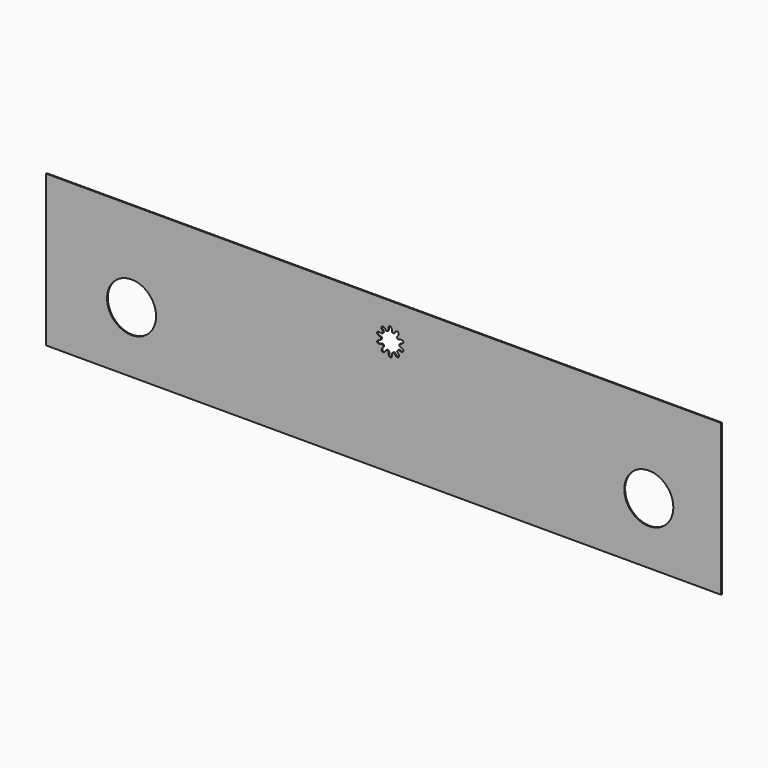
from build123d import *

# Parameters (mm, degrees)
F0_W     = 89.1250632703
F0_H     = 19.9663289823
F0_R     = 3.235221554
F1_DEPTH = 0.127


# Not quite as in the source:
# - ends of sketch curves that miss each other by under 0.0002 mm in the source are joined


with BuildPart() as f1:
    # F0 (on Front) → F1 (new body)
    with BuildSketch(Plane.XZ):
        with Locations((-0.8681025356, -5.2086075302)):
            Rectangle(F0_W, F0_H)
        with Locations((-34.1453179717, -7.0894937962)):
            Circle(F0_R, mode=Mode.SUBTRACT)
        with Locations((34.1453179717, -7.0894937962)):
            Circle(F0_R, mode=Mode.SUBTRACT)
        with BuildLine():
            Line((0.638931, 1.307427), (0.642386, 1.31177))
            Line((0.642386, 1.31177), (0.645946, 1.316251))
            Line((0.645946, 1.316251), (0.649602, 1.320915))
            Line((0.649602, 1.320915), (0.653347, 1.325811))
            Line((0.653347, 1.325811), (0.657176, 1.330987))
            Line((0.657176, 1.330987), (0.66108, 1.336491))
            Line((0.66108, 1.336491), (0.665063, 1.34235))
            Line((0.665063, 1.34235), (0.66917, 1.34852))
            Line((0.66917, 1.34852), (0.673459, 1.354933))
            Line((0.673459, 1.354933), (0.677985, 1.361525))
            Line((0.677985, 1.361525), (0.682804, 1.368231))
            Line((0.682804, 1.368231), (0.687974, 1.374984))
            Line((0.687974, 1.374984), (0.693549, 1.38172))
            Line((0.693549, 1.38172), (0.699587, 1.388373))
            Line((0.699587, 1.388373), (0.706145, 1.394901))
            Line((0.706145, 1.394901), (0.713282, 1.401347))
            Line((0.713282, 1.401347), (0.721059, 1.407781))
            Line((0.721059, 1.407781), (0.729537, 1.41427))
            Line((0.729537, 1.41427), (0.738776, 1.420881))
            Line((0.738776, 1.420881), (0.748838, 1.427684))
            Line((0.748838, 1.427684), (0.759782, 1.434744))
            Line((0.759782, 1.434744), (0.771669, 1.44213))
            Line((0.771669, 1.44213), (0.784656, 1.449932))
            Line((0.784656, 1.449932), (0.799284, 1.458325))
            Line((0.799284, 1.458325), (0.816191, 1.467508))
            Line((0.816191, 1.467508), (0.836013, 1.477679))
            Line((0.836013, 1.477679), (0.859387, 1.489035))
            Line((0.859387, 1.489035), (0.886951, 1.501775))
            Line((0.886951, 1.501775), (0.919341, 1.516097))
            Line((0.919341, 1.516097), (0.949649, 1.528989))
            ThreePointArc((0.949649, 1.528989), (1.0419801318, 1.4676230494), (1.1303581966, 1.4006892437))
            Line((1.1303581966, 1.4006892437), (1.128181, 1.367826))
            Line((1.128181, 1.367826), (1.12534, 1.332524))
            Line((1.12534, 1.332524), (1.122401, 1.302301))
            Line((1.122401, 1.302301), (1.119386, 1.27649))
            Line((1.119386, 1.27649), (1.11632, 1.254423))
            Line((1.11632, 1.254423), (1.113225, 1.235434))
            Line((1.113225, 1.235434), (1.110125, 1.218856))
            Line((1.110125, 1.218856), (1.107041, 1.204023))
            Line((1.107041, 1.204023), (1.103988, 1.190365))
            Line((1.103988, 1.190365), (1.100931, 1.177705))
            Line((1.100931, 1.177705), (1.097827, 1.165964))
            Line((1.097827, 1.165964), (1.094631, 1.155061))
            Line((1.094631, 1.155061), (1.091301, 1.144918))
            Line((1.091301, 1.144918), (1.087791, 1.135454))
            Line((1.087791, 1.135454), (1.084058, 1.126591))
            Line((1.084058, 1.126591), (1.080058, 1.118248))
            Line((1.080058, 1.118248), (1.075768, 1.110353))
            Line((1.075768, 1.110353), (1.071247, 1.102868))
            Line((1.071247, 1.102868), (1.066576, 1.095761))
            Line((1.066576, 1.095761), (1.061834, 1.089))
            Line((1.061834, 1.089), (1.057103, 1.082554))
            Line((1.057103, 1.082554), (1.052463, 1.07639))
            Line((1.052463, 1.07639), (1.047993, 1.070478))
            Line((1.047993, 1.070478), (1.043774, 1.064786))
            Line((1.043774, 1.064786), (1.039866, 1.059286))
            Line((1.039866, 1.059286), (1.036242, 1.053965))
            Line((1.036242, 1.053965), (1.032854, 1.048814))
            Line((1.032854, 1.048814), (1.029656, 1.043825))
            Line((1.029656, 1.043825), (1.0266, 1.038987))
            Line((1.0266, 1.038987), (1.023639, 1.034293))
            Line((1.023639, 1.034293), (1.020725, 1.029733))
            Line((1.020725, 1.029733), (1.017811, 1.025298))
            Line((1.017811, 1.025298), (1.014863, 1.020986))
            Line((1.014863, 1.020986), (1.011898, 1.016826))
            Line((1.011898, 1.016826), (1.008947, 1.012851))
            Line((1.008947, 1.012851), (1.00604, 1.009097))
            Line((1.00604, 1.009097), (1.003207, 1.005598))
            Line((1.003207, 1.005598), (1.00048, 1.00239))
            Line((1.00048, 1.00239), (0.997889, 0.999506))
            Line((0.997889, 0.999506), (0.995464, 0.996983))
            Line((0.995464, 0.996983), (0.918412, 0.888456))
            ThreePointArc((0.918412, 0.888456), (0.900022697, 0.8267789399), (0.9230261025, 0.7666700851))
            ThreePointArc((0.9230261025, 0.7666700851), (0.9629750976, 0.7158484276), (1.0001292142, 0.662949142))
            ThreePointArc((1.0001292142, 0.662949142), (1.0510595113, 0.6236013113), (1.115418799, 0.6234375965))
            Line((1.115418799, 0.6234375965), (1.241546, 0.665948))
            Line((1.241546, 0.665948), (1.244661, 0.667543))
            Line((1.244661, 0.667543), (1.248169, 0.669193))
            Line((1.248169, 0.669193), (1.252027, 0.67088))
            Line((1.252027, 0.67088), (1.256194, 0.672584))
            Line((1.256194, 0.672584), (1.260626, 0.674286))
            Line((1.260626, 0.674286), (1.265283, 0.675967))
            Line((1.265283, 0.675967), (1.270122, 0.677607))
            Line((1.270122, 0.677607), (1.2751, 0.679188))
            Line((1.2751, 0.679188), (1.280186, 0.6807))
            Line((1.280186, 0.6807), (1.285393, 0.682176))
            Line((1.285393, 0.682176), (1.290741, 0.683659))
            Line((1.290741, 0.683659), (1.296254, 0.685192))
            Line((1.296254, 0.685192), (1.301953, 0.686816))
            Line((1.301953, 0.686816), (1.307862, 0.688576))
            Line((1.307862, 0.688576), (1.314001, 0.690513))
            Line((1.314001, 0.690513), (1.320394, 0.692671))
            Line((1.320394, 0.692671), (1.327061, 0.69507))
            Line((1.327061, 0.69507), (1.33401, 0.697647))
            Line((1.33401, 0.697647), (1.341249, 0.700315))
            Line((1.341249, 0.700315), (1.348786, 0.702987))
            Line((1.348786, 0.702987), (1.356626, 0.70558))
            Line((1.356626, 0.70558), (1.364778, 0.708005))
            Line((1.364778, 0.708005), (1.373248, 0.710177))
            Line((1.373248, 0.710177), (1.382044, 0.71201))
            Line((1.382044, 0.71201), (1.391186, 0.713437))
            Line((1.391186, 0.713437), (1.400749, 0.714457))
            Line((1.400749, 0.714457), (1.410822, 0.715091))
            Line((1.410822, 0.715091), (1.421495, 0.715357))
            Line((1.421495, 0.715357), (1.432856, 0.715275))
            Line((1.432856, 0.715275), (1.444994, 0.714864))
            Line((1.444994, 0.714864), (1.457998, 0.714144))
            Line((1.457998, 0.714144), (1.471956, 0.713132))
            Line((1.471956, 0.713132), (1.487049, 0.71181))
            Line((1.487049, 0.71181), (1.503817, 0.710002))
            Line((1.503817, 0.710002), (1.522892, 0.707494))
            Line((1.522892, 0.707494), (1.544906, 0.704071))
            Line((1.544906, 0.704071), (1.570492, 0.69952))
            Line((1.570492, 0.69952), (1.60028, 0.693625))
            Line((1.60028, 0.693625), (1.634903, 0.686173))
            Line((1.634903, 0.686173), (1.666999, 0.678788))
            ThreePointArc((1.666999, 0.678788), (1.7056267642, 0.5748715955), (1.7377833197, 0.4687740862))
            Line((1.7377833197, 0.4687740862), (1.716705, 0.443466))
            Line((1.716705, 0.443466), (1.693657, 0.416577))
            Line((1.693657, 0.416577), (1.673515, 0.393853))
            Line((1.673515, 0.393853), (1.655905, 0.374743))
            Line((1.655905, 0.374743), (1.640453, 0.358693))
            Line((1.640453, 0.358693), (1.626788, 0.34515))
            Line((1.626788, 0.34515), (1.614536, 0.33356))
            Line((1.614536, 0.33356), (1.603322, 0.323372))
            Line((1.603322, 0.323372), (1.592824, 0.314118))
            Line((1.592824, 0.314118), (1.58291, 0.305672))
            Line((1.58291, 0.305672), (1.573497, 0.297998))
            Line((1.573497, 0.297998), (1.564503, 0.291056))
            Line((1.564503, 0.291056), (1.555847, 0.284807))
            Line((1.555847, 0.284807), (1.547445, 0.279214))
            Line((1.547445, 0.279214), (1.539215, 0.274237))
            Line((1.539215, 0.274237), (1.531075, 0.269839))
            Line((1.531075, 0.269839), (1.522964, 0.265974))
            Line((1.522964, 0.265974), (1.514907, 0.262576))
            Line((1.514907, 0.262576), (1.506951, 0.259572))
            Line((1.506951, 0.259572), (1.499141, 0.256889))
            Line((1.499141, 0.256889), (1.491524, 0.254455))
            Line((1.491524, 0.254455), (1.484147, 0.252196))
            Line((1.484147, 0.252196), (1.477056, 0.25004))
            Line((1.477056, 0.25004), (1.470297, 0.247915))
            Line((1.470297, 0.247915), (1.463902, 0.245763))
            Line((1.463902, 0.245763), (1.457842, 0.243588))
            Line((1.457842, 0.243588), (1.452074, 0.241412))
            Line((1.452074, 0.241412), (1.446554, 0.239255))
            Line((1.446554, 0.239255), (1.441238, 0.237138))
            Line((1.441238, 0.237138), (1.436084, 0.235081))
            Line((1.436084, 0.235081), (1.431046, 0.233104))
            Line((1.431046, 0.233104), (1.426082, 0.231229))
            Line((1.426082, 0.231229), (1.421162, 0.229474))
            Line((1.421162, 0.229474), (1.416318, 0.227851))
            Line((1.416318, 0.227851), (1.411594, 0.22637))
            Line((1.411594, 0.22637), (1.407036, 0.225041))
            Line((1.407036, 0.225041), (1.402688, 0.223875))
            Line((1.402688, 0.223875), (1.398596, 0.222883))
            Line((1.398596, 0.222883), (1.394804, 0.222073))
            Line((1.394804, 0.222073), (1.391359, 0.221457))
            Line((1.391359, 0.221457), (1.265232, 0.178947))
            ThreePointArc((1.265232, 0.178947), (1.214102181, 0.1398577938), (1.1973809136, 0.0777079944))
            ThreePointArc((1.1973809136, 0.0777079944), (1.1998283673, 0.013111024), (1.1987932625, -0.0515240113))
            ThreePointArc((1.1987932625, -0.0515240113), (1.2168684266, -0.1132934724), (1.2688401361, -0.151255565))
            Line((1.2688401361, -0.151255565), (1.395867, -0.191))
            Line((1.395867, -0.191), (1.399324, -0.19154))
            Line((1.399324, -0.19154), (1.403132, -0.192267))
            Line((1.403132, -0.192267), (1.407245, -0.19317))
            Line((1.407245, -0.19317), (1.411618, -0.19424))
            Line((1.411618, -0.19424), (1.416204, -0.195469))
            Line((1.416204, -0.195469), (1.420959, -0.196846))
            Line((1.420959, -0.196846), (1.425838, -0.198363))
            Line((1.425838, -0.198363), (1.430794, -0.20001))
            Line((1.430794, -0.20001), (1.435798, -0.201777))
            Line((1.435798, -0.201777), (1.440878, -0.203643))
            Line((1.440878, -0.203643), (1.446076, -0.205587))
            Line((1.446076, -0.205587), (1.451437, -0.207587))
            Line((1.451437, -0.207587), (1.457003, -0.209623))
            Line((1.457003, -0.209623), (1.462817, -0.211672))
            Line((1.462817, -0.211672), (1.468923, -0.213714))
            Line((1.468923, -0.213714), (1.475363, -0.215726))
            Line((1.475363, -0.215726), (1.482167, -0.217703))
            Line((1.482167, -0.217703), (1.489304, -0.219703))
            Line((1.489304, -0.219703), (1.496728, -0.2218))
            Line((1.496728, -0.2218), (1.504396, -0.224068))
            Line((1.504396, -0.224068), (1.512263, -0.226579))
            Line((1.512263, -0.226579), (1.520284, -0.229409))
            Line((1.520284, -0.229409), (1.528413, -0.23263))
            Line((1.528413, -0.23263), (1.536606, -0.236316))
            Line((1.536606, -0.236316), (1.54484, -0.240536))
            Line((1.54484, -0.240536), (1.553177, -0.245332))
            Line((1.553177, -0.245332), (1.561699, -0.25074))
            Line((1.561699, -0.25074), (1.57049, -0.256798))
            Line((1.57049, -0.256798), (1.579633, -0.263542))
            Line((1.579633, -0.263542), (1.589212, -0.271009))
            Line((1.589212, -0.271009), (1.599308, -0.279235))
            Line((1.599308, -0.279235), (1.610006, -0.288258))
            Line((1.610006, -0.288258), (1.621439, -0.298199))
            Line((1.621439, -0.298199), (1.633942, -0.309518))
            Line((1.633942, -0.309518), (1.6479, -0.322759))
            Line((1.6479, -0.322759), (1.663698, -0.338468))
            Line((1.663698, -0.338468), (1.681722, -0.357189))
            Line((1.681722, -0.357189), (1.702356, -0.379466))
            Line((1.702356, -0.379466), (1.725987, -0.405846))
            Line((1.725987, -0.405846), (1.747612, -0.430686))
            ThreePointArc((1.747612, -0.430686), (1.717782042, -0.5374615021), (1.6814345016, -0.6421978097))
            Line((1.6814345016, -0.6421978097), (1.649507, -0.650282))
            Line((1.649507, -0.650282), (1.615055, -0.658489))
            Line((1.615055, -0.658489), (1.585403, -0.665033))
            Line((1.585403, -0.665033), (1.559924, -0.670143))
            Line((1.559924, -0.670143), (1.537989, -0.674046))
            Line((1.537989, -0.674046), (1.518973, -0.67697))
            Line((1.518973, -0.67697), (1.502249, -0.679144))
            Line((1.502249, -0.679144), (1.487189, -0.680796))
            Line((1.487189, -0.680796), (1.473256, -0.682112))
            Line((1.473256, -0.682112), (1.460271, -0.683117))
            Line((1.460271, -0.683117), (1.448145, -0.683793))
            Line((1.448145, -0.683793), (1.436788, -0.684123))
            Line((1.436788, -0.684123), (1.426112, -0.68409))
            Line((1.426112, -0.68409), (1.416027, -0.683676))
            Line((1.416027, -0.683676), (1.406444, -0.682865))
            Line((1.406444, -0.682865), (1.397273, -0.681639))
            Line((1.397273, -0.681639), (1.38844, -0.679999))
            Line((1.38844, -0.679999), (1.379924, -0.678012))
            Line((1.379924, -0.678012), (1.371721, -0.675765))
            Line((1.371721, -0.675765), (1.363826, -0.673345))
            Line((1.363826, -0.673345), (1.356233, -0.670838))
            Line((1.356233, -0.670838), (1.348937, -0.668329))
            Line((1.348937, -0.668329), (1.341933, -0.665905))
            Line((1.341933, -0.665905), (1.335216, -0.663652))
            Line((1.335216, -0.663652), (1.328777, -0.661634))
            Line((1.328777, -0.661634), (1.322597, -0.659831))
            Line((1.322597, -0.659831), (1.316651, -0.658201))
            Line((1.316651, -0.658201), (1.310918, -0.656702))
            Line((1.310918, -0.656702), (1.305373, -0.65529))
            Line((1.305373, -0.65529), (1.299993, -0.653924))
            Line((1.299993, -0.653924), (1.294756, -0.652562))
            Line((1.294756, -0.652562), (1.289638, -0.651162))
            Line((1.289638, -0.651162), (1.284626, -0.64969))
            Line((1.284626, -0.64969), (1.279753, -0.648156))
            Line((1.279753, -0.648156), (1.275061, -0.646577))
            Line((1.275061, -0.646577), (1.270592, -0.644973))
            Line((1.270592, -0.644973), (1.266389, -0.64336))
            Line((1.266389, -0.64336), (1.262495, -0.641758))
            Line((1.262495, -0.641758), (1.258952, -0.640185))
            Line((1.258952, -0.640185), (1.255803, -0.638658))
            Line((1.255803, -0.638658), (1.128777, -0.598914))
            ThreePointArc((1.128777, -0.598914), (1.0644359855, -0.6004833879), (1.0143773054, -0.6409355611))
            ThreePointArc((1.0143773054, -0.6409355611), (0.9783880245, -0.6946343524), (0.9395589449, -0.7463169562))
            ThreePointArc((0.9395589449, -0.7463169562), (0.9178748171, -0.8069139849), (0.9376076019, -0.8681742959))
            Line((0.9376076019, -0.8681742959), (1.017013, -0.974992))
            Line((1.017013, -0.974992), (1.019493, -0.977462))
            Line((1.019493, -0.977462), (1.022147, -0.980288))
            Line((1.022147, -0.980288), (1.024943, -0.983436))
            Line((1.024943, -0.983436), (1.027851, -0.986872))
            Line((1.027851, -0.986872), (1.03084, -0.990561))
            Line((1.03084, -0.990561), (1.033877, -0.994471))
            Line((1.033877, -0.994471), (1.036932, -0.998566))
            Line((1.036932, -0.998566), (1.039974, -1.002812))
            Line((1.039974, -1.002812), (1.042984, -1.007182))
            Line((1.042984, -1.007182), (1.045997, -1.011677))
            Line((1.045997, -1.011677), (1.04906, -1.016306))
            Line((1.04906, -1.016306), (1.052221, -1.021075))
            Line((1.052221, -1.021075), (1.055527, -1.025993))
            Line((1.055527, -1.025993), (1.059026, -1.031069))
            Line((1.059026, -1.031069), (1.062766, -1.036309))
            Line((1.062766, -1.036309), (1.066794, -1.041723))
            Line((1.066794, -1.041723), (1.071136, -1.047322))
            Line((1.071136, -1.047322), (1.075734, -1.053135))
            Line((1.075734, -1.053135), (1.080508, -1.059195))
            Line((1.080508, -1.059195), (1.085379, -1.065537))
            Line((1.085379, -1.065537), (1.090267, -1.072192))
            Line((1.090267, -1.072192), (1.095092, -1.079196))
            Line((1.095092, -1.079196), (1.099776, -1.08658))
            Line((1.099776, -1.08658), (1.104238, -1.094379))
            Line((1.104238, -1.094379), (1.108419, -1.102632))
            Line((1.108419, -1.102632), (1.112344, -1.111412))
            Line((1.112344, -1.111412), (1.11606, -1.120797))
            Line((1.11606, -1.120797), (1.119612, -1.130865))
            Line((1.119612, -1.130865), (1.123044, -1.141695))
            Line((1.123044, -1.141695), (1.126404, -1.153366))
            Line((1.126404, -1.153366), (1.129737, -1.165956))
            Line((1.129737, -1.165956), (1.133089, -1.179544))
            Line((1.133089, -1.179544), (1.136495, -1.194306))
            Line((1.136495, -1.194306), (1.139957, -1.210812))
            Line((1.139957, -1.210812), (1.143467, -1.229729))
            Line((1.143467, -1.229729), (1.147014, -1.251724))
            Line((1.147014, -1.251724), (1.150592, -1.277463))
            Line((1.150592, -1.277463), (1.154191, -1.307615))
            Line((1.154191, -1.307615), (1.157802, -1.342846))
            Line((1.157802, -1.342846), (1.160697, -1.375654))
            ThreePointArc((1.160697, -1.375654), (1.0738028266, -1.4445025094), (0.9828350637, -1.5078710978))
            Line((0.9828350637, -1.5078710978), (0.952253, -1.495645))
            Line((0.952253, -1.495645), (0.919557, -1.482035))
            Line((0.919557, -1.482035), (0.891722, -1.4699))
            Line((0.891722, -1.4699), (0.868105, -1.459057))
            Line((0.868105, -1.459057), (0.848065, -1.449322))
            Line((0.848065, -1.449322), (0.830962, -1.440511))
            Line((0.830962, -1.440511), (0.816154, -1.432439))
            Line((0.816154, -1.432439), (0.802999, -1.424923))
            Line((0.802999, -1.424923), (0.790954, -1.417798))
            Line((0.790954, -1.417798), (0.779858, -1.410979))
            Line((0.779858, -1.410979), (0.769651, -1.404398))
            Line((0.769651, -1.404398), (0.760269, -1.39799))
            Line((0.760269, -1.39799), (0.751651, -1.391688))
            Line((0.751651, -1.391688), (0.743736, -1.385426))
            Line((0.743736, -1.385426), (0.736459, -1.379137))
            Line((0.736459, -1.379137), (0.729761, -1.372755))
            Line((0.729761, -1.372755), (0.723578, -1.366235))
            Line((0.723578, -1.366235), (0.717857, -1.359622))
            Line((0.717857, -1.359622), (0.712541, -1.352983))
            Line((0.712541, -1.352983), (0.707576, -1.346385))
            Line((0.707576, -1.346385), (0.702907, -1.339893))
            Line((0.702907, -1.339893), (0.69848, -1.333575))
            Line((0.69848, -1.333575), (0.694238, -1.327497))
            Line((0.694238, -1.327497), (0.690128, -1.321726))
            Line((0.690128, -1.321726), (0.686105, -1.316309))
            Line((0.686105, -1.316309), (0.682164, -1.311218))
            Line((0.682164, -1.311218), (0.678313, -1.306404))
            Line((0.678313, -1.306404), (0.674555, -1.301821))
            Line((0.674555, -1.301821), (0.670899, -1.29742))
            Line((0.670899, -1.29742), (0.66735, -1.293153))
            Line((0.66735, -1.293153), (0.663913, -1.288973))
            Line((0.663913, -1.288973), (0.660596, -1.284831))
            Line((0.660596, -1.284831), (0.657406, -1.280695))
            Line((0.657406, -1.280695), (0.654366, -1.276589))
            Line((0.654366, -1.276589), (0.651497, -1.272554))
            Line((0.651497, -1.272554), (0.648825, -1.268629))
            Line((0.648825, -1.268629), (0.646373, -1.264854))
            Line((0.646373, -1.264854), (0.644164, -1.261269))
            Line((0.644164, -1.261269), (0.642223, -1.257914))
            Line((0.642223, -1.257914), (0.640572, -1.254828))
            Line((0.640572, -1.254828), (0.561167, -1.14801))
            ThreePointArc((0.561167, -1.14801), (0.508191214, -1.1114617005), (0.4439160796, -1.1147641999))
            ThreePointArc((0.4439160796, -1.1147641999), (0.3832371001, -1.1370529166), (0.32144593, -1.1560417484))
            ThreePointArc((0.32144593, -1.1560417484), (0.2682848788, -1.1923205525), (0.2482409734, -1.2534800003))
            Line((0.2482409734, -1.2534800003), (0.249695, -1.38657))
            Line((0.249695, -1.38657), (0.25025, -1.390026))
            Line((0.25025, -1.390026), (0.250736, -1.393872))
            Line((0.250736, -1.393872), (0.251148, -1.398063))
            Line((0.251148, -1.398063), (0.251481, -1.402552))
            Line((0.251481, -1.402552), (0.25173, -1.407293))
            Line((0.25173, -1.407293), (0.251889, -1.412242))
            Line((0.251889, -1.412242), (0.251954, -1.41735))
            Line((0.251954, -1.41735), (0.251919, -1.422573))
            Line((0.251919, -1.422573), (0.251785, -1.427878))
            Line((0.251785, -1.427878), (0.251581, -1.433286))
            Line((0.251581, -1.433286), (0.251338, -1.43883))
            Line((0.251338, -1.43883), (0.251092, -1.444547))
            Line((0.251092, -1.444547), (0.250876, -1.45047))
            Line((0.250876, -1.45047), (0.250723, -1.456633))
            Line((0.250723, -1.456633), (0.250669, -1.46307))
            Line((0.250669, -1.46307), (0.250745, -1.469817))
            Line((0.250745, -1.469817), (0.250967, -1.476899))
            Line((0.250967, -1.476899), (0.25127, -1.484304))
            Line((0.25127, -1.484304), (0.25157, -1.492014))
            Line((0.25157, -1.492014), (0.251783, -1.500007))
            Line((0.251783, -1.500007), (0.251826, -1.508265))
            Line((0.251826, -1.508265), (0.251613, -1.516767))
            Line((0.251613, -1.516767), (0.251062, -1.525494))
            Line((0.251062, -1.525494), (0.250088, -1.534426))
            Line((0.250088, -1.534426), (0.248619, -1.543561))
            Line((0.248619, -1.543561), (0.246634, -1.552971))
            Line((0.246634, -1.552971), (0.244124, -1.562748))
            Line((0.244124, -1.562748), (0.241079, -1.57298))
            Line((0.241079, -1.57298), (0.237491, -1.58376))
            Line((0.237491, -1.58376), (0.233349, -1.595177))
            Line((0.233349, -1.595177), (0.228645, -1.607321))
            Line((0.228645, -1.607321), (0.22337, -1.620284))
            Line((0.22337, -1.620284), (0.217449, -1.634229))
            Line((0.217449, -1.634229), (0.210548, -1.649618))
            Line((0.210548, -1.649618), (0.202268, -1.666984))
            Line((0.202268, -1.666984), (0.19221, -1.686864))
            Line((0.19221, -1.686864), (0.179975, -1.70979))
            Line((0.179975, -1.70979), (0.165163, -1.736299))
            Line((0.165163, -1.736299), (0.147377, -1.766924))
            Line((0.147377, -1.766924), (0.130435, -1.795168))
            ThreePointArc((0.130435, -1.795168), (0.0196678117, -1.79979254), (-0.0911739649, -1.7975893074))
            Line((-0.0911739649, -1.7975893074), (-0.108729, -1.769723))
            Line((-0.108729, -1.769723), (-0.127181, -1.739494))
            Line((-0.127181, -1.739494), (-0.142567, -1.713315))
            Line((-0.142567, -1.713315), (-0.155301, -1.690661))
            Line((-0.155301, -1.690661), (-0.165791, -1.671007))
            Line((-0.165791, -1.671007), (-0.174448, -1.653825))
            Line((-0.174448, -1.653825), (-0.181684, -1.638591))
            Line((-0.181684, -1.638591), (-0.187908, -1.624778))
            Line((-0.187908, -1.624778), (-0.193466, -1.611934))
            Line((-0.193466, -1.611934), (-0.198434, -1.599895))
            Line((-0.198434, -1.599895), (-0.202824, -1.588572))
            Line((-0.202824, -1.588572), (-0.206647, -1.577873))
            Line((-0.206647, -1.577873), (-0.209915, -1.567709))
            Line((-0.209915, -1.567709), (-0.212638, -1.55799))
            Line((-0.212638, -1.55799), (-0.214828, -1.548625))
            Line((-0.214828, -1.548625), (-0.216496, -1.539524))
            Line((-0.216496, -1.539524), (-0.217665, -1.530616))
            Line((-0.217665, -1.530616), (-0.218407, -1.521903))
            Line((-0.218407, -1.521903), (-0.218805, -1.513408))
            Line((-0.218805, -1.513408), (-0.218944, -1.505151))
            Line((-0.218944, -1.505151), (-0.218905, -1.497155))
            Line((-0.218905, -1.497155), (-0.218774, -1.489441))
            Line((-0.218774, -1.489441), (-0.218632, -1.482031))
            Line((-0.218632, -1.482031), (-0.218565, -1.474946))
            Line((-0.218565, -1.474946), (-0.218636, -1.468199))
            Line((-0.218636, -1.468199), (-0.218832, -1.461764))
            Line((-0.218832, -1.461764), (-0.219119, -1.455606))
            Line((-0.219119, -1.455606), (-0.219464, -1.449689))
            Line((-0.219464, -1.449689), (-0.219835, -1.443979))
            Line((-0.219835, -1.443979), (-0.220199, -1.438441))
            Line((-0.220199, -1.438441), (-0.220522, -1.433039))
            Line((-0.220522, -1.433039), (-0.220771, -1.427739))
            Line((-0.220771, -1.427739), (-0.22092, -1.422518))
            Line((-0.22092, -1.422518), (-0.220967, -1.417409))
            Line((-0.220967, -1.417409), (-0.220916, -1.412458))
            Line((-0.220916, -1.412458), (-0.220771, -1.407713))
            Line((-0.220771, -1.407713), (-0.220536, -1.403217))
            Line((-0.220536, -1.403217), (-0.220215, -1.399019))
            Line((-0.220215, -1.399019), (-0.219814, -1.395163))
            Line((-0.219814, -1.395163), (-0.219335, -1.391696))
            Line((-0.219335, -1.391696), (-0.220789, -1.258605))
            ThreePointArc((-0.220789, -1.258605), (-0.2421648006, -1.1978984957), (-0.2961059025, -1.1627906171))
            ThreePointArc((-0.2961059025, -1.1627906171), (-0.3582973113, -1.1451563416), (-0.4194488769, -1.12419867))
            ThreePointArc((-0.4194488769, -1.12419867), (-0.4837808515, -1.1223017261), (-0.5359450962, -1.1599989317))
            Line((-0.5359450962, -1.1599989317), (-0.612998, -1.268526))
            Line((-0.612998, -1.268526), (-0.61458, -1.271648))
            Line((-0.61458, -1.271648), (-0.616448, -1.275045))
            Line((-0.616448, -1.275045), (-0.618578, -1.278677))
            Line((-0.618578, -1.278677), (-0.620947, -1.282505))
            Line((-0.620947, -1.282505), (-0.623533, -1.286487))
            Line((-0.623533, -1.286487), (-0.626312, -1.290584))
            Line((-0.626312, -1.290584), (-0.629262, -1.294755))
            Line((-0.629262, -1.294755), (-0.632361, -1.29896))
            Line((-0.632361, -1.29896), (-0.635587, -1.303173))
            Line((-0.635587, -1.303173), (-0.638931, -1.307428))
            Line((-0.638931, -1.307428), (-0.642386, -1.311771))
            Line((-0.642386, -1.311771), (-0.645946, -1.316251))
            Line((-0.645946, -1.316251), (-0.649602, -1.320916))
            Line((-0.649602, -1.320916), (-0.653347, -1.325812))
            Line((-0.653347, -1.325812), (-0.657176, -1.330988))
            Line((-0.657176, -1.330988), (-0.66108, -1.336492))
            Line((-0.66108, -1.336492), (-0.665063, -1.342351))
            Line((-0.665063, -1.342351), (-0.66917, -1.34852))
            Line((-0.66917, -1.34852), (-0.673459, -1.354934))
            Line((-0.673459, -1.354934), (-0.677985, -1.361526))
            Line((-0.677985, -1.361526), (-0.682804, -1.368231))
            Line((-0.682804, -1.368231), (-0.687974, -1.374985))
            Line((-0.687974, -1.374985), (-0.693549, -1.381721))
            Line((-0.693549, -1.381721), (-0.699587, -1.388374))
            Line((-0.699587, -1.388374), (-0.706145, -1.394901))
            Line((-0.706145, -1.394901), (-0.713282, -1.401348))
            Line((-0.713282, -1.401348), (-0.721059, -1.407782))
            Line((-0.721059, -1.407782), (-0.729537, -1.414271))
            Line((-0.729537, -1.414271), (-0.738776, -1.420882))
            Line((-0.738776, -1.420882), (-0.748838, -1.427684))
            Line((-0.748838, -1.427684), (-0.759782, -1.434744))
            Line((-0.759782, -1.434744), (-0.771669, -1.442131))
            Line((-0.771669, -1.442131), (-0.784656, -1.449932))
            Line((-0.784656, -1.449932), (-0.799284, -1.458326))
            Line((-0.799284, -1.458326), (-0.816191, -1.467509))
            Line((-0.816191, -1.467509), (-0.836013, -1.47768))
            Line((-0.836013, -1.47768), (-0.859387, -1.489036))
            Line((-0.859387, -1.489036), (-0.886951, -1.501776))
            Line((-0.886951, -1.501776), (-0.919341, -1.516098))
            Line((-0.919341, -1.516098), (-0.949649, -1.528989))
            ThreePointArc((-0.949649, -1.528989), (-1.0419798757, -1.4676232311), (-1.1303577079, -1.4006896381))
            Line((-1.1303577079, -1.4006896381), (-1.128181, -1.367827))
            Line((-1.128181, -1.367827), (-1.12534, -1.332525))
            Line((-1.12534, -1.332525), (-1.122401, -1.302302))
            Line((-1.122401, -1.302302), (-1.119386, -1.27649))
            Line((-1.119386, -1.27649), (-1.11632, -1.254424))
            Line((-1.11632, -1.254424), (-1.113225, -1.235435))
            Line((-1.113225, -1.235435), (-1.110125, -1.218857))
            Line((-1.110125, -1.218857), (-1.107041, -1.204024))
            Line((-1.107041, -1.204024), (-1.103988, -1.190366))
            Line((-1.103988, -1.190366), (-1.100931, -1.177706))
            Line((-1.100931, -1.177706), (-1.097827, -1.165964))
            Line((-1.097827, -1.165964), (-1.094631, -1.155062))
            Line((-1.094631, -1.155062), (-1.091301, -1.144919))
            Line((-1.091301, -1.144919), (-1.087791, -1.135455))
            Line((-1.087791, -1.135455), (-1.084058, -1.126591))
            Line((-1.084058, -1.126591), (-1.080058, -1.118248))
            Line((-1.080058, -1.118248), (-1.075768, -1.110354))
            Line((-1.075768, -1.110354), (-1.071247, -1.102869))
            Line((-1.071247, -1.102869), (-1.066576, -1.095762))
            Line((-1.066576, -1.095762), (-1.061834, -1.089001))
            Line((-1.061834, -1.089001), (-1.057103, -1.082555))
            Line((-1.057103, -1.082555), (-1.052463, -1.076391))
            Line((-1.052463, -1.076391), (-1.047993, -1.070479))
            Line((-1.047993, -1.070479), (-1.043774, -1.064787))
            Line((-1.043774, -1.064787), (-1.039866, -1.059287))
            Line((-1.039866, -1.059287), (-1.036242, -1.053966))
            Line((-1.036242, -1.053966), (-1.032854, -1.048815))
            Line((-1.032854, -1.048815), (-1.029656, -1.043825))
            Line((-1.029656, -1.043825), (-1.0266, -1.038988))
            Line((-1.0266, -1.038988), (-1.023639, -1.034294))
            Line((-1.023639, -1.034294), (-1.020725, -1.029734))
            Line((-1.020725, -1.029734), (-1.017811, -1.025299))
            Line((-1.017811, -1.025299), (-1.014863, -1.020987))
            Line((-1.014863, -1.020987), (-1.011898, -1.016827))
            Line((-1.011898, -1.016827), (-1.008947, -1.012852))
            Line((-1.008947, -1.012852), (-1.00604, -1.009098))
            Line((-1.00604, -1.009098), (-1.003207, -1.005599))
            Line((-1.003207, -1.005599), (-1.00048, -1.00239))
            Line((-1.00048, -1.00239), (-0.997889, -0.999507))
            Line((-0.997889, -0.999507), (-0.995464, -0.996984))
            Line((-0.995464, -0.996984), (-0.918412, -0.888456))
            ThreePointArc((-0.918412, -0.888456), (-0.9000226824, -0.8267793243), (-0.923025611, -0.7666706769))
            ThreePointArc((-0.923025611, -0.7666706769), (-0.9629746195, -0.7158490708), (-1.0001287537, -0.6629498367))
            ThreePointArc((-1.0001287537, -0.6629498367), (-1.0510592681, -0.6236013946), (-1.1154191016, -0.6234376985))
            Line((-1.1154191016, -0.6234376985), (-1.241546, -0.665949))
            Line((-1.241546, -0.665949), (-1.244661, -0.667544))
            Line((-1.244661, -0.667544), (-1.248169, -0.669194))
            Line((-1.248169, -0.669194), (-1.252027, -0.670881))
            Line((-1.252027, -0.670881), (-1.256194, -0.672585))
            Line((-1.256194, -0.672585), (-1.260627, -0.674287))
            Line((-1.260627, -0.674287), (-1.265283, -0.675968))
            Line((-1.265283, -0.675968), (-1.270122, -0.677608))
            Line((-1.270122, -0.677608), (-1.2751, -0.679189))
            Line((-1.2751, -0.679189), (-1.280186, -0.680701))
            Line((-1.280186, -0.680701), (-1.285393, -0.682177))
            Line((-1.285393, -0.682177), (-1.290741, -0.68366))
            Line((-1.290741, -0.68366), (-1.296254, -0.685192))
            Line((-1.296254, -0.685192), (-1.301953, -0.686817))
            Line((-1.301953, -0.686817), (-1.307862, -0.688577))
            Line((-1.307862, -0.688577), (-1.314001, -0.690514))
            Line((-1.314001, -0.690514), (-1.320395, -0.692672))
            Line((-1.320395, -0.692672), (-1.327061, -0.695071))
            Line((-1.327061, -0.695071), (-1.33401, -0.697648))
            Line((-1.33401, -0.697648), (-1.341249, -0.700315))
            Line((-1.341249, -0.700315), (-1.348786, -0.702988))
            Line((-1.348786, -0.702988), (-1.356626, -0.70558))
            Line((-1.356626, -0.70558), (-1.364778, -0.708005))
            Line((-1.364778, -0.708005), (-1.373248, -0.710178))
            Line((-1.373248, -0.710178), (-1.382044, -0.712011))
            Line((-1.382044, -0.712011), (-1.391186, -0.713437))
            Line((-1.391186, -0.713437), (-1.400749, -0.714458))
            Line((-1.400749, -0.714458), (-1.410822, -0.715091))
            Line((-1.410822, -0.715091), (-1.421495, -0.715358))
            Line((-1.421495, -0.715358), (-1.432856, -0.715276))
            Line((-1.432856, -0.715276), (-1.444994, -0.714865))
            Line((-1.444994, -0.714865), (-1.457998, -0.714144))
            Line((-1.457998, -0.714144), (-1.471956, -0.713133))
            Line((-1.471956, -0.713133), (-1.487049, -0.711811))
            Line((-1.487049, -0.711811), (-1.503817, -0.710003))
            Line((-1.503817, -0.710003), (-1.522892, -0.707495))
            Line((-1.522892, -0.707495), (-1.544906, -0.704072))
            Line((-1.544906, -0.704072), (-1.570492, -0.699521))
            Line((-1.570492, -0.699521), (-1.60028, -0.693626))
            Line((-1.60028, -0.693626), (-1.634903, -0.686174))
            Line((-1.634903, -0.686174), (-1.666999, -0.678789))
            ThreePointArc((-1.666999, -0.678789), (-1.7056266163, -0.5748720344), (-1.7377833197, -0.4687740862))
            Line((-1.7377833197, -0.4687740862), (-1.716705, -0.443467))
            Line((-1.716705, -0.443467), (-1.693657, -0.416577))
            Line((-1.693657, -0.416577), (-1.673515, -0.393854))
            Line((-1.673515, -0.393854), (-1.655905, -0.374744))
            Line((-1.655905, -0.374744), (-1.640453, -0.358693))
            Line((-1.640453, -0.358693), (-1.626788, -0.34515))
            Line((-1.626788, -0.34515), (-1.614536, -0.333561))
            Line((-1.614536, -0.333561), (-1.603322, -0.323373))
            Line((-1.603322, -0.323373), (-1.592824, -0.314118))
            Line((-1.592824, -0.314118), (-1.58291, -0.305673))
            Line((-1.58291, -0.305673), (-1.573497, -0.297999))
            Line((-1.573497, -0.297999), (-1.564504, -0.291057))
            Line((-1.564504, -0.291057), (-1.555847, -0.284808))
            Line((-1.555847, -0.284808), (-1.547445, -0.279215))
            Line((-1.547445, -0.279215), (-1.539215, -0.274238))
            Line((-1.539215, -0.274238), (-1.531075, -0.26984))
            Line((-1.531075, -0.26984), (-1.522964, -0.265975))
            Line((-1.522964, -0.265975), (-1.514907, -0.262577))
            Line((-1.514907, -0.262577), (-1.506951, -0.259573))
            Line((-1.506951, -0.259573), (-1.499141, -0.25689))
            Line((-1.499141, -0.25689), (-1.491524, -0.254455))
            Line((-1.491524, -0.254455), (-1.484147, -0.252197))
            Line((-1.484147, -0.252197), (-1.477056, -0.250041))
            Line((-1.477056, -0.250041), (-1.470297, -0.247916))
            Line((-1.470297, -0.247916), (-1.463902, -0.245763))
            Line((-1.463902, -0.245763), (-1.457842, -0.243589))
            Line((-1.457842, -0.243589), (-1.452074, -0.241413))
            Line((-1.452074, -0.241413), (-1.446554, -0.239256))
            Line((-1.446554, -0.239256), (-1.441239, -0.237139))
            Line((-1.441239, -0.237139), (-1.436084, -0.235082))
            Line((-1.436084, -0.235082), (-1.431046, -0.233105))
            Line((-1.431046, -0.233105), (-1.426082, -0.23123))
            Line((-1.426082, -0.23123), (-1.421162, -0.229475))
            Line((-1.421162, -0.229475), (-1.416318, -0.227851))
            Line((-1.416318, -0.227851), (-1.411594, -0.22637))
            Line((-1.411594, -0.22637), (-1.407036, -0.225042))
            Line((-1.407036, -0.225042), (-1.402688, -0.223876))
            Line((-1.402688, -0.223876), (-1.398596, -0.222883))
            Line((-1.398596, -0.222883), (-1.394804, -0.222074))
            Line((-1.394804, -0.222074), (-1.391359, -0.221458))
            Line((-1.391359, -0.221458), (-1.265232, -0.178947))
            ThreePointArc((-1.265232, -0.178947), (-1.2141020921, -0.1398586612), (-1.1973809136, -0.0777089944))
            ThreePointArc((-1.1973809136, -0.0777089944), (-1.1998283564, -0.0131120224), (-1.1987933054, 0.0515230131))
            ThreePointArc((-1.1987933054, 0.0515230131), (-1.2168684266, 0.1132924724), (-1.2688401361, 0.151254565))
            Line((-1.2688401361, 0.151254565), (-1.395867, 0.190999))
            Line((-1.395867, 0.190999), (-1.399324, 0.191539))
            Line((-1.399324, 0.191539), (-1.403132, 0.192266))
            Line((-1.403132, 0.192266), (-1.407245, 0.193169))
            Line((-1.407245, 0.193169), (-1.411618, 0.194239))
            Line((-1.411618, 0.194239), (-1.416204, 0.195468))
            Line((-1.416204, 0.195468), (-1.420959, 0.196845))
            Line((-1.420959, 0.196845), (-1.425838, 0.198362))
            Line((-1.425838, 0.198362), (-1.430794, 0.20001))
            Line((-1.430794, 0.20001), (-1.435798, 0.201776))
            Line((-1.435798, 0.201776), (-1.440878, 0.203642))
            Line((-1.440878, 0.203642), (-1.446077, 0.205586))
            Line((-1.446077, 0.205586), (-1.451437, 0.207586))
            Line((-1.451437, 0.207586), (-1.457003, 0.209622))
            Line((-1.457003, 0.209622), (-1.462817, 0.211672))
            Line((-1.462817, 0.211672), (-1.468923, 0.213713))
            Line((-1.468923, 0.213713), (-1.475364, 0.215725))
            Line((-1.475364, 0.215725), (-1.482167, 0.217702))
            Line((-1.482167, 0.217702), (-1.489304, 0.219703))
            Line((-1.489304, 0.219703), (-1.496728, 0.2218))
            Line((-1.496728, 0.2218), (-1.504396, 0.224067))
            Line((-1.504396, 0.224067), (-1.512263, 0.226578))
            Line((-1.512263, 0.226578), (-1.520284, 0.229408))
            Line((-1.520284, 0.229408), (-1.528413, 0.232629))
            Line((-1.528413, 0.232629), (-1.536606, 0.236316))
            Line((-1.536606, 0.236316), (-1.54484, 0.240535))
            Line((-1.54484, 0.240535), (-1.553177, 0.245331))
            Line((-1.553177, 0.245331), (-1.561699, 0.250739))
            Line((-1.561699, 0.250739), (-1.57049, 0.256797))
            Line((-1.57049, 0.256797), (-1.579633, 0.263541))
            Line((-1.579633, 0.263541), (-1.589212, 0.271008))
            Line((-1.589212, 0.271008), (-1.599308, 0.279235))
            Line((-1.599308, 0.279235), (-1.610006, 0.288257))
            Line((-1.610006, 0.288257), (-1.621439, 0.298198))
            Line((-1.621439, 0.298198), (-1.633942, 0.309517))
            Line((-1.633942, 0.309517), (-1.6479, 0.322758))
            Line((-1.6479, 0.322758), (-1.663698, 0.338467))
            Line((-1.663698, 0.338467), (-1.681722, 0.357188))
            Line((-1.681722, 0.357188), (-1.702356, 0.379466))
            Line((-1.702356, 0.379466), (-1.725987, 0.405845))
            Line((-1.725987, 0.405845), (-1.747613, 0.430686))
            ThreePointArc((-1.747613, 0.430686), (-1.7177822172, 0.5374609421), (-1.6814348349, 0.642196937))
            Line((-1.6814348349, 0.642196937), (-1.649507, 0.650282))
            Line((-1.649507, 0.650282), (-1.615056, 0.658489))
            Line((-1.615056, 0.658489), (-1.585403, 0.665033))
            Line((-1.585403, 0.665033), (-1.559924, 0.670142))
            Line((-1.559924, 0.670142), (-1.537989, 0.674045))
            Line((-1.537989, 0.674045), (-1.518973, 0.67697))
            Line((-1.518973, 0.67697), (-1.502249, 0.679143))
            Line((-1.502249, 0.679143), (-1.487189, 0.680795))
            Line((-1.487189, 0.680795), (-1.473256, 0.682111))
            Line((-1.473256, 0.682111), (-1.460271, 0.683116))
            Line((-1.460271, 0.683116), (-1.448145, 0.683792))
            Line((-1.448145, 0.683792), (-1.436789, 0.684122))
            Line((-1.436789, 0.684122), (-1.426112, 0.684089))
            Line((-1.426112, 0.684089), (-1.416027, 0.683676))
            Line((-1.416027, 0.683676), (-1.406444, 0.682865))
            Line((-1.406444, 0.682865), (-1.397273, 0.681639))
            Line((-1.397273, 0.681639), (-1.38844, 0.679998))
            Line((-1.38844, 0.679998), (-1.379924, 0.678011))
            Line((-1.379924, 0.678011), (-1.371721, 0.675765))
            Line((-1.371721, 0.675765), (-1.363826, 0.673345))
            Line((-1.363826, 0.673345), (-1.356233, 0.670837))
            Line((-1.356233, 0.670837), (-1.348937, 0.668328))
            Line((-1.348937, 0.668328), (-1.341933, 0.665904))
            Line((-1.341933, 0.665904), (-1.335216, 0.663651))
            Line((-1.335216, 0.663651), (-1.328777, 0.661633))
            Line((-1.328777, 0.661633), (-1.322597, 0.659831))
            Line((-1.322597, 0.659831), (-1.316651, 0.658201))
            Line((-1.316651, 0.658201), (-1.310918, 0.656701))
            Line((-1.310918, 0.656701), (-1.305373, 0.655289))
            Line((-1.305373, 0.655289), (-1.299993, 0.653924))
            Line((-1.299993, 0.653924), (-1.294756, 0.652562))
            Line((-1.294756, 0.652562), (-1.289638, 0.651161))
            Line((-1.289638, 0.651161), (-1.284626, 0.649689))
            Line((-1.284626, 0.649689), (-1.279753, 0.648155))
            Line((-1.279753, 0.648155), (-1.275061, 0.646577))
            Line((-1.275061, 0.646577), (-1.270592, 0.644972))
            Line((-1.270592, 0.644972), (-1.266389, 0.643359))
            Line((-1.266389, 0.643359), (-1.262495, 0.641757))
            Line((-1.262495, 0.641757), (-1.258952, 0.640184))
            Line((-1.258952, 0.640184), (-1.255803, 0.638657))
            Line((-1.255803, 0.638657), (-1.128777, 0.598913))
            ThreePointArc((-1.128777, 0.598913), (-1.0644362421, 0.6004832936), (-1.014377757, 0.6409348464))
            ThreePointArc((-1.014377757, 0.6409348464), (-0.9783884958, 0.6946336885), (-0.9395594319, 0.7463163431))
            ThreePointArc((-0.9395594319, 0.7463163431), (-0.9178758169, 0.8069129976), (-0.937608246, 0.8681728171))
            Line((-0.937608246, 0.8681728171), (-1.017013, 0.974991))
            Line((-1.017013, 0.974991), (-1.019493, 0.977461))
            Line((-1.019493, 0.977461), (-1.022147, 0.980287))
            Line((-1.022147, 0.980287), (-1.024943, 0.983435))
            Line((-1.024943, 0.983435), (-1.027851, 0.986871))
            Line((-1.027851, 0.986871), (-1.03084, 0.990561))
            Line((-1.03084, 0.990561), (-1.033877, 0.99447))
            Line((-1.033877, 0.99447), (-1.036932, 0.998565))
            Line((-1.036932, 0.998565), (-1.039974, 1.002811))
            Line((-1.039974, 1.002811), (-1.042984, 1.007181))
            Line((-1.042984, 1.007181), (-1.045997, 1.011676))
            Line((-1.045997, 1.011676), (-1.04906, 1.016305))
            Line((-1.04906, 1.016305), (-1.052221, 1.021074))
            Line((-1.052221, 1.021074), (-1.055527, 1.025993))
            Line((-1.055527, 1.025993), (-1.059026, 1.031068))
            Line((-1.059026, 1.031068), (-1.062766, 1.036309))
            Line((-1.062766, 1.036309), (-1.066794, 1.041722))
            Line((-1.066794, 1.041722), (-1.071136, 1.047321))
            Line((-1.071136, 1.047321), (-1.075734, 1.053134))
            Line((-1.075734, 1.053134), (-1.080508, 1.059194))
            Line((-1.080508, 1.059194), (-1.085379, 1.065536))
            Line((-1.085379, 1.065536), (-1.090267, 1.072192))
            Line((-1.090267, 1.072192), (-1.095092, 1.079195))
            Line((-1.095092, 1.079195), (-1.099776, 1.086579))
            Line((-1.099776, 1.086579), (-1.104238, 1.094378))
            Line((-1.104238, 1.094378), (-1.108419, 1.102632))
            Line((-1.108419, 1.102632), (-1.112344, 1.111411))
            Line((-1.112344, 1.111411), (-1.11606, 1.120796))
            Line((-1.11606, 1.120796), (-1.119612, 1.130864))
            Line((-1.119612, 1.130864), (-1.123044, 1.141694))
            Line((-1.123044, 1.141694), (-1.126404, 1.153365))
            Line((-1.126404, 1.153365), (-1.129737, 1.165955))
            Line((-1.129737, 1.165955), (-1.133089, 1.179543))
            Line((-1.133089, 1.179543), (-1.136495, 1.194305))
            Line((-1.136495, 1.194305), (-1.139957, 1.210811))
            Line((-1.139957, 1.210811), (-1.143467, 1.229728))
            Line((-1.143467, 1.229728), (-1.147014, 1.251723))
            Line((-1.147014, 1.251723), (-1.150592, 1.277462))
            Line((-1.150592, 1.277462), (-1.154191, 1.307614))
            Line((-1.154191, 1.307614), (-1.157802, 1.342845))
            Line((-1.157802, 1.342845), (-1.160697, 1.375653))
            ThreePointArc((-1.160697, 1.375653), (-1.0738030854, 1.444502317), (-0.9828350637, 1.5078710978))
            Line((-0.9828350637, 1.5078710978), (-0.952253, 1.495645))
            Line((-0.952253, 1.495645), (-0.919557, 1.482034))
            Line((-0.919557, 1.482034), (-0.891722, 1.469899))
            Line((-0.891722, 1.469899), (-0.868105, 1.459056))
            Line((-0.868105, 1.459056), (-0.848065, 1.449321))
            Line((-0.848065, 1.449321), (-0.830962, 1.44051))
            Line((-0.830962, 1.44051), (-0.816154, 1.432438))
            Line((-0.816154, 1.432438), (-0.803, 1.424922))
            Line((-0.803, 1.424922), (-0.790954, 1.417798))
            Line((-0.790954, 1.417798), (-0.779858, 1.410978))
            Line((-0.779858, 1.410978), (-0.769651, 1.404398))
            Line((-0.769651, 1.404398), (-0.760269, 1.39799))
            Line((-0.760269, 1.39799), (-0.751651, 1.391688))
            Line((-0.751651, 1.391688), (-0.743736, 1.385425))
            Line((-0.743736, 1.385425), (-0.736459, 1.379136))
            Line((-0.736459, 1.379136), (-0.729761, 1.372754))
            Line((-0.729761, 1.372754), (-0.723578, 1.366234))
            Line((-0.723578, 1.366234), (-0.717857, 1.359621))
            Line((-0.717857, 1.359621), (-0.712541, 1.352983))
            Line((-0.712541, 1.352983), (-0.707576, 1.346384))
            Line((-0.707576, 1.346384), (-0.702907, 1.339892))
            Line((-0.702907, 1.339892), (-0.69848, 1.333574))
            Line((-0.69848, 1.333574), (-0.694238, 1.327496))
            Line((-0.694238, 1.327496), (-0.690128, 1.321725))
            Line((-0.690128, 1.321725), (-0.686105, 1.316308))
            Line((-0.686105, 1.316308), (-0.682164, 1.311217))
            Line((-0.682164, 1.311217), (-0.678313, 1.306404))
            Line((-0.678313, 1.306404), (-0.674555, 1.30182))
            Line((-0.674555, 1.30182), (-0.670899, 1.297419))
            Line((-0.670899, 1.297419), (-0.66735, 1.293152))
            Line((-0.66735, 1.293152), (-0.663913, 1.288972))
            Line((-0.663913, 1.288972), (-0.660596, 1.28483))
            Line((-0.660596, 1.28483), (-0.657406, 1.280694))
            Line((-0.657406, 1.280694), (-0.654366, 1.276588))
            Line((-0.654366, 1.276588), (-0.651497, 1.272553))
            Line((-0.651497, 1.272553), (-0.648825, 1.268628))
            Line((-0.648825, 1.268628), (-0.646373, 1.264854))
            Line((-0.646373, 1.264854), (-0.644164, 1.261268))
            Line((-0.644164, 1.261268), (-0.642223, 1.257913))
            Line((-0.642223, 1.257913), (-0.640572, 1.254827))
            Line((-0.640572, 1.254827), (-0.561167, 1.148009))
            ThreePointArc((-0.561167, 1.148009), (-0.508191214, 1.1114607005), (-0.4439160796, 1.1147631999))
            ThreePointArc((-0.4439160796, 1.1147631999), (-0.3832374023, 1.1370528147), (-0.3214461881, 1.1560416766))
            ThreePointArc((-0.3214461881, 1.1560416766), (-0.2682848788, 1.1923195525), (-0.2482409734, 1.2534790003))
            Line((-0.2482409734, 1.2534790003), (-0.249695, 1.38657))
            Line((-0.249695, 1.38657), (-0.25025, 1.390025))
            Line((-0.25025, 1.390025), (-0.250736, 1.393871))
            Line((-0.250736, 1.393871), (-0.251148, 1.398062))
            Line((-0.251148, 1.398062), (-0.251481, 1.402551))
            Line((-0.251481, 1.402551), (-0.25173, 1.407293))
            Line((-0.25173, 1.407293), (-0.251889, 1.412241))
            Line((-0.251889, 1.412241), (-0.251954, 1.417349))
            Line((-0.251954, 1.417349), (-0.251919, 1.422572))
            Line((-0.251919, 1.422572), (-0.251785, 1.427877))
            Line((-0.251785, 1.427877), (-0.251581, 1.433285))
            Line((-0.251581, 1.433285), (-0.251338, 1.43883))
            Line((-0.251338, 1.43883), (-0.251092, 1.444546))
            Line((-0.251092, 1.444546), (-0.250876, 1.450469))
            Line((-0.250876, 1.450469), (-0.250723, 1.456632))
            Line((-0.250723, 1.456632), (-0.250669, 1.46307))
            Line((-0.250669, 1.46307), (-0.250745, 1.469817))
            Line((-0.250745, 1.469817), (-0.250967, 1.476898))
            Line((-0.250967, 1.476898), (-0.25127, 1.484304))
            Line((-0.25127, 1.484304), (-0.25157, 1.492013))
            Line((-0.25157, 1.492013), (-0.251784, 1.500006))
            Line((-0.251784, 1.500006), (-0.251826, 1.508264))
            Line((-0.251826, 1.508264), (-0.251613, 1.516766))
            Line((-0.251613, 1.516766), (-0.251062, 1.525493))
            Line((-0.251062, 1.525493), (-0.250088, 1.534425))
            Line((-0.250088, 1.534425), (-0.248619, 1.54356))
            Line((-0.248619, 1.54356), (-0.246634, 1.55297))
            Line((-0.246634, 1.55297), (-0.244124, 1.562747))
            Line((-0.244124, 1.562747), (-0.241079, 1.57298))
            Line((-0.241079, 1.57298), (-0.237491, 1.583759))
            Line((-0.237491, 1.583759), (-0.233349, 1.595176))
            Line((-0.233349, 1.595176), (-0.228645, 1.60732))
            Line((-0.228645, 1.60732), (-0.22337, 1.620283))
            Line((-0.22337, 1.620283), (-0.217449, 1.634228))
            Line((-0.217449, 1.634228), (-0.210548, 1.649617))
            Line((-0.210548, 1.649617), (-0.202268, 1.666984))
            Line((-0.202268, 1.666984), (-0.19221, 1.686863))
            Line((-0.19221, 1.686863), (-0.179975, 1.70979))
            Line((-0.179975, 1.70979), (-0.165163, 1.736298))
            Line((-0.165163, 1.736298), (-0.147377, 1.766924))
            Line((-0.147377, 1.766924), (-0.130435, 1.795167))
            ThreePointArc((-0.130435, 1.795167), (-0.0196678226, 1.7997925399), (0.0911740155, 1.7975893048))
            Line((0.0911740155, 1.7975893048), (0.108729, 1.769722))
            Line((0.108729, 1.769722), (0.127181, 1.739493))
            Line((0.127181, 1.739493), (0.142567, 1.713314))
            Line((0.142567, 1.713314), (0.155301, 1.690661))
            Line((0.155301, 1.690661), (0.165791, 1.671006))
            Line((0.165791, 1.671006), (0.174448, 1.653824))
            Line((0.174448, 1.653824), (0.181684, 1.63859))
            Line((0.181684, 1.63859), (0.187908, 1.624778))
            Line((0.187908, 1.624778), (0.193466, 1.611933))
            Line((0.193466, 1.611933), (0.198434, 1.599894))
            Line((0.198434, 1.599894), (0.202824, 1.588571))
            Line((0.202824, 1.588571), (0.206647, 1.577872))
            Line((0.206647, 1.577872), (0.209915, 1.567708))
            Line((0.209915, 1.567708), (0.212638, 1.557989))
            Line((0.212638, 1.557989), (0.214828, 1.548624))
            Line((0.214828, 1.548624), (0.216496, 1.539524))
            Line((0.216496, 1.539524), (0.217665, 1.530615))
            Line((0.217665, 1.530615), (0.218407, 1.521903))
            Line((0.218407, 1.521903), (0.218805, 1.513407))
            Line((0.218805, 1.513407), (0.218944, 1.50515))
            Line((0.218944, 1.50515), (0.218905, 1.497154))
            Line((0.218905, 1.497154), (0.218773, 1.48944))
            Line((0.218773, 1.48944), (0.218632, 1.48203))
            Line((0.218632, 1.48203), (0.218565, 1.474945))
            Line((0.218565, 1.474945), (0.218636, 1.468198))
            Line((0.218636, 1.468198), (0.218832, 1.461763))
            Line((0.218832, 1.461763), (0.219119, 1.455605))
            Line((0.219119, 1.455605), (0.219464, 1.449688))
            Line((0.219464, 1.449688), (0.219835, 1.443979))
            Line((0.219835, 1.443979), (0.220199, 1.43844))
            Line((0.220199, 1.43844), (0.220522, 1.433038))
            Line((0.220522, 1.433038), (0.220771, 1.427738))
            Line((0.220771, 1.427738), (0.22092, 1.422517))
            Line((0.22092, 1.422517), (0.220967, 1.417408))
            Line((0.220967, 1.417408), (0.220916, 1.412458))
            Line((0.220916, 1.412458), (0.220771, 1.407712))
            Line((0.220771, 1.407712), (0.220536, 1.403216))
            Line((0.220536, 1.403216), (0.220215, 1.399018))
            Line((0.220215, 1.399018), (0.219814, 1.395162))
            Line((0.219814, 1.395162), (0.219335, 1.391695))
            Line((0.219335, 1.391695), (0.220789, 1.258604))
            ThreePointArc((0.220789, 1.258604), (0.2421648006, 1.1978974957), (0.2961059025, 1.1627896171))
            ThreePointArc((0.2961059025, 1.1627896171), (0.3582975959, 1.1451562526), (0.4194492044, 1.1241985478))
            ThreePointArc((0.4194492044, 1.1241985478), (0.4837808515, 1.1223007261), (0.5359450962, 1.1599979317))
            Line((0.5359450962, 1.1599979317), (0.612998, 1.268526))
            Line((0.612998, 1.268526), (0.61458, 1.271647))
            Line((0.61458, 1.271647), (0.616448, 1.275044))
            Line((0.616448, 1.275044), (0.618578, 1.278677))
            Line((0.618578, 1.278677), (0.620947, 1.282504))
            Line((0.620947, 1.282504), (0.623533, 1.286487))
            Line((0.623533, 1.286487), (0.626312, 1.290583))
            Line((0.626312, 1.290583), (0.629262, 1.294754))
            Line((0.629262, 1.294754), (0.632361, 1.298959))
            Line((0.632361, 1.298959), (0.635587, 1.303173))
            Line((0.635587, 1.303173), (0.638931, 1.307427))
        make_face(mode=Mode.SUBTRACT)
    extrude(amount=F1_DEPTH)


solid = f1.part
